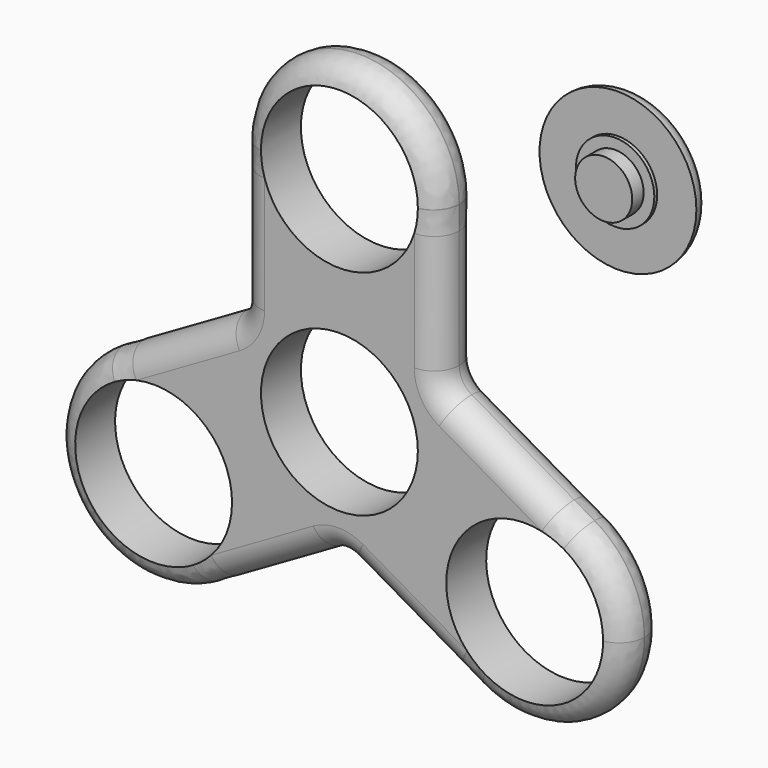
from build123d import *

# Parameters (mm, degrees)
F0_R     = 11
F1_DEPTH = 7
F2_R     = 11
F2_R_2   = 5.5
F3_DEPTH = 2.5
F2_R_3   = 4
F4_DEPTH = 3
F5_DEPTH = 5
F6_R     = 3.49999
F7_R     = 2.49999


# Not quite as in the source:
# - a fillet or chamfer is up to 0.001 mm smaller than in the source, because OpenCascade refuses the exact size


with BuildPart() as f1:
    # F0 (on Front) → F1 (new body)
    with BuildSketch(Plane.XZ):
        with BuildLine():
            Line((-14, 15), (-14, -6.7050106472))
            Line((-14, -6.7050106472), (-33.0630497308, -17.7110675409))
            ThreePointArc((-33.0630497308, -17.7110675409), (-38.1874053838, -36.8354231939), (-19.0630497308, -41.9597788469))
            Line((-19.0630497308, -41.9597788469), (-0.1836715036, -31.0597647453))
            Line((-0.1836715036, -31.0597647453), (18.9807621135, -42.124355653))
            ThreePointArc((18.9807621135, -42.124355653), (38.1051177665, -37), (32.9807621135, -17.875644347))
            Line((32.9807621135, -17.875644347), (14, -6.9170962313))
            Line((14, -6.9170962313), (14, 15))
            ThreePointArc((14, 15), (0, 29), (-14, 15))
        make_face()
        with Locations((-26.0630497308, -29.8354231939)):
            Circle(F0_R, mode=Mode.SUBTRACT)
        with Locations((25.9807621135, -30)):
            Circle(F0_R, mode=Mode.SUBTRACT)
        with Locations((0, -15)):
            Circle(F0_R, mode=Mode.SUBTRACT)
        with Locations((0, 15)):
            Circle(F0_R, mode=Mode.SUBTRACT)
    extrude(amount=F1_DEPTH)

    # F6 (radius 3.5 in the source; OpenCascade refuses exactly that, so slightly less here)
    f6_edges = [f1.edges().sort_by_distance(p)[0] for p in [
        (-14, -3.5, 15),
        (-14, -3.5, -6.705011),
        (-14, 0, 4.147495),
        (-14, -7, 4.147495),
        (-33.06305, -3.5, -17.711068),
        (-23.531525, 0, -12.208039),
        (-23.531525, -7, -12.208039),
        (-19.06305, -3.5, -41.959779),
        (-38.187405, 0, -36.835423),
        (-38.187405, -7, -36.835423),
        (14, -3.5, 15),
        (0, 0, 29),
        (0, -7, 29),
        (-0.183672, -3.5, -31.059765),
        (-9.623361, 0, -36.509772),
        (-9.623361, -7, -36.509772),
        (18.980762, -3.5, -42.124356),
        (32.980762, -3.5, -17.875644),
        (38.105118, 0, -37),
        (38.105118, -7, -37),
        (9.398545, 0, -36.59206),
        (9.398545, -7, -36.59206),
        (14, -3.5, -6.917096),
        (23.490381, 0, -12.39637),
        (23.490381, -7, -12.39637),
        (14, 0, 4.041452),
        (14, -7, 4.041452),
    ]]
    fillet(f6_edges, radius=F6_R)


with BuildPart() as f3:
    # F2 (on Front) → F3 (new body)
    with BuildSketch(Plane.XZ):
        with Locations((35.4663021863, 24.5219450444)):
            Circle(F2_R)
        with Locations((35.4663021863, 24.5219450444)):
            Circle(F2_R_2, mode=Mode.SUBTRACT)
    extrude(amount=F3_DEPTH)

    # F2 (on Front) → F4 (join)
    with BuildSketch(Plane.XZ):
        with Locations((35.4663021863, 24.5219450444)):
            Circle(F2_R_2)
        with Locations((35.4663021863, 24.5219450444)):
            Circle(F2_R_3, mode=Mode.SUBTRACT)
    extrude(amount=F4_DEPTH)

    # F2 (on Front) → F5 (join)
    with BuildSketch(Plane.XZ):
        with Locations((35.4663021863, 24.5219450444)):
            Circle(F2_R_3)
    extrude(amount=F5_DEPTH)

    # F7 (radius 2.5 in the source; OpenCascade refuses exactly that, so slightly less here)
    f7_edges = [f3.edges().sort_by_distance(p)[0] for p in [
        (24.466302, 0, 24.521945),
    ]]
    fillet(f7_edges, radius=F7_R)


solid = Compound([f1.part, f3.part])
